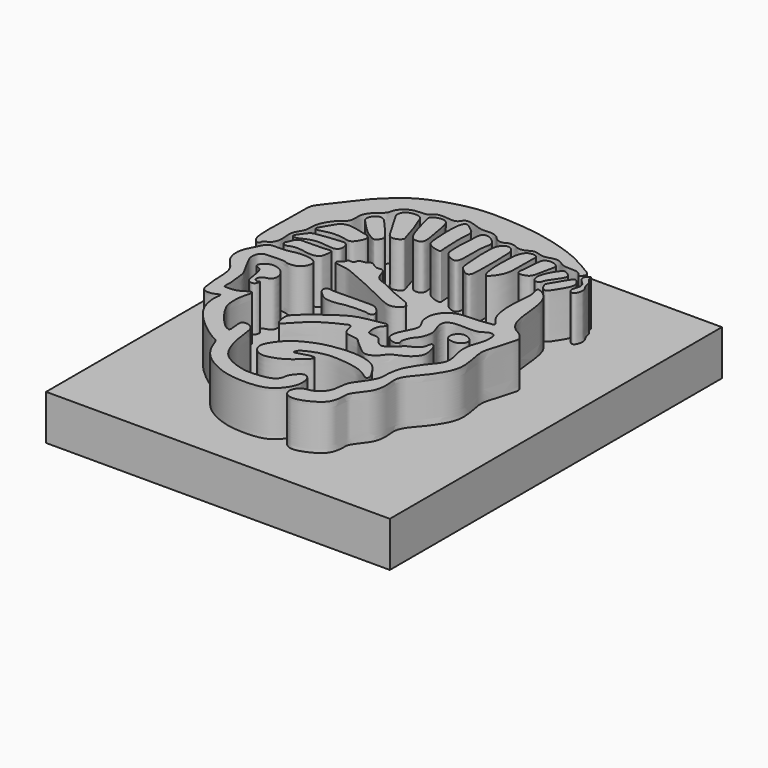
from build123d import *

# Parameters (mm, degrees)
F1_DEPTH = 25.4
F2_W     = 96.9264013693
F2_H     = 117.0432046056
F3_DEPTH = 12.7


with BuildPart() as f1:
    # F0 (on Top) → F1 (new body)
    with BuildSketch(Plane.XY):
        with BuildLine():
            add(Edge.make_bspline(
                [(-40.2134470642, -13.6436549947), (-40.5038319253, -13.0532989312), (-40.9712662134, -12.0357692788), (-40.3828119426, -9.0838404135), (-37.4700159523, -9.1659597907), (-33.6801272021, -8.8772320002), (-32.7655772786, -9.6282652278), (-29.8023894039, -9.4210274483), (-28.3806589854, -7.5498569946), (-28.0532124759, -5.5301169959), (-29.9501063345, -4.2010879959), (-33.9584884018, -4.060553572), (-36.4882191847, -4.9901386676), (-39.7344326102, -4.8370794081), (-41.852988261, -5.0813649106), (-43.0611123611, -7.9930232863), (-44.6638586961, -10.8148641524), (-44.6805787942, -13.9824924027), (-43.4351839453, -16.5508592113), (-41.4060540395, -18.327504016), (-40.4817112793, -20.4170340166), (-40.2150456125, -23.173487216), (-40.2371317705, -25.6148272624), (-39.7897618651, -28.8111673703), (-39.4242040094, -31.1359618698), (-36.7206525589, -31.2192672972), (-35.6066458214, -30.6210898454), (-34.4127301406, -30.0990799373), (-34.932395965, -32.2774129262), (-34.6889736884, -34.3855625988), (-33.9514081898, -37.3805205335), (-31.9389951827, -40.3046677573), (-29.0667186094, -43.1618199647), (-26.052819601, -45.5593423485), (-23.5900655555, -47.2267415521), (-21.6999075012, -47.8249153248), (-21.0648357224, -50.7700427907), (-18.8106721799, -54.2710823292), (-15.7050192032, -56.747814972), (-10.9850909536, -58.9656562044), (-5.5210704614, -59.6254274225), (0.0655429157, -59.2721168152), (3.1418643476, -57.3279514264), (5.3379892447, -54.0854350072), (5.6011670768, -51.5204836423), (5.2429584174, -49.3374778631), (3.4009534995, -48.166607769), (1.8703771285, -49.6207679802), (0.6615174644, -51.2282183426), (0.7409672686, -52.993382624), (-0.928557497, -54.7108114083), (-4.556009372, -55.1621405529), (-8.4581184608, -55.3892312796), (-13.3437110299, -53.5718738684), (-15.8033997352, -51.6433831739), (-17.4804730559, -48.8032608251), (-18.6647319579, -44.6349468246), (-19.0353626337, -40.8983524571), (-19.4757454842, -38.3228496413), (-21.5701928172, -37.2608658786), (-23.1594355454, -37.7347875195), (-22.9633855567, -39.5685823373), (-22.5875095291, -42.186811965), (-23.232268811, -42.0865318242), (-24.1233688412, -41.7328370024), (-25.2311286943, -40.8741082801), (-28.213025083, -37.5769037551), (-30.2068242336, -34.1381189549), (-30.7460865655, -32.4917857606), (-30.7936590907, -28.9726861151), (-30.1021813845, -26.3503756002), (-29.7493093459, -25.166157434), (-30.5926807443, -24.9813323567), (-31.6427370917, -25.773252658), (-33.4709586463, -26.8433998571), (-36.2557679667, -26.8237017314), (-36.7498527526, -26.6771194484), (-36.4617540337, -24.7653587113), (-37.0026261542, -21.1625112292), (-37.1052353815, -19.1935704677), (-38.8213673131, -16.3662075654), (-39.8354152195, -14.4121984746), (-40.2134470642, -13.6436549947)],
                knots=[0, 0, 0, 0, 0.0105854357, 0.0227038139, 0.0355615522, 0.0506964042, 0.0590934994, 0.0718715099, 0.08372586, 0.0940838712, 0.1051368075, 0.1206855449, 0.1338879249, 0.147872312, 0.1586917055, 0.1720366682, 0.1864080274, 0.2000583123, 0.2131788584, 0.2259198188, 0.2376677544, 0.2505637198, 0.2630490339, 0.2772986456, 0.2884688624, 0.3002440343, 0.3096215137, 0.3164567212, 0.3264983543, 0.3384916292, 0.3520782106, 0.3668620136, 0.3827581289, 0.3983550294, 0.4118200351, 0.4221569994, 0.4351815037, 0.4512043984, 0.4668630146, 0.4845956824, 0.503265583, 0.5216125929, 0.5364037424, 0.5516107261, 0.5641673247, 0.5755537169, 0.5858159785, 0.5965098416, 0.6076312106, 0.6176334598, 0.6290166971, 0.6438033901, 0.6596293721, 0.6773473823, 0.691109071, 0.7051053782, 0.7215553422, 0.7369683211, 0.7492434926, 0.7605774012, 0.769367475, 0.7798612926, 0.7919744263, 0.7966216104, 0.8041149769, 0.8133299168, 0.8300412854, 0.8457482662, 0.8560105345, 0.8706321915, 0.8839702758, 0.8916090014, 0.8975101119, 0.9062586889, 0.9181242245, 0.9309764693, 0.9355028424, 0.9456931412, 0.9609607679, 0.972097378, 0.9862195579, 1, 1, 1, 1], degree=3))
        make_face()
        with BuildLine():
            add(Edge.make_bspline(
                [(-36.9890481234, 1.9141569501), (-37.6086093115, 1.6183880837), (-38.5317237833, 1.0516364801), (-40.4055938126, 1.3458247704), (-38.8954202479, 3.4409428718), (-37.7142225728, 5.0654187852), (-36.2422882152, 5.4533680411), (-31.0847105816, 6.0055868791), (-29.4042524296, 6.2039104022), (-28.1776089982, 6.0259950489), (-27.4019390923, 3.5957598157), (-28.6162726688, 2.2319888659), (-30.9662986649, 2.5583398946), (-34.3116035087, 2.9699572864), (-36.2321994637, 2.2754647181), (-36.9890481234, 1.9141569501)],
                knots=[0, 0, 0, 0, 0.072612367, 0.129661764, 0.2048222141, 0.2807607212, 0.345890099, 0.4667093526, 0.5374814039, 0.5905759148, 0.6694874813, 0.7336228202, 0.8127819433, 0.9112975866, 1, 1, 1, 1], degree=3))
        make_face()
    extrude(amount=F1_DEPTH)



with BuildPart() as f1b:
    # F0 (on Top) → F1, piece 2 (new body)
    with BuildSketch(Plane.XY):
        with BuildLine():
            add(Edge.make_bspline(
                [(-35.3266075253, -16.0623975098), (-35.4972584298, -15.6958523644), (-35.9577022635, -15.0490288372), (-37.1653320579, -14.8763550547), (-37.4622378024, -13.8763719918), (-35.9694428669, -12.2011305597), (-33.6958844721, -12.0077739228), (-31.3642934169, -13.1003837915), (-29.9891050699, -15.3295362371), (-30.5140421494, -17.6267172637), (-32.215666586, -17.7794257093), (-33.1899626709, -18.4639808352), (-33.6363150575, -19.8373776846), (-32.2927485056, -20.601676247), (-31.836702742, -19.6812009092), (-31.7990430425, -21.0156581463), (-32.6426422962, -21.8861025724), (-34.3389047052, -21.358790101), (-34.6550812728, -19.4363616515), (-34.8919011587, -17.4700956508), (-35.1363620882, -16.471030219), (-35.3266075253, -16.0623975098)],
                knots=[0, 0, 0, 0, 0.0473231751, 0.0931074818, 0.1316273518, 0.193737266, 0.2588862114, 0.3280781791, 0.3976259368, 0.4589092763, 0.5125312499, 0.5600258653, 0.6082496238, 0.6549574763, 0.6858732626, 0.7261825163, 0.7726873443, 0.8248430499, 0.8843108095, 0.9472430682, 1, 1, 1, 1], degree=3))
        make_face()
    extrude(amount=F1_DEPTH)


with BuildPart() as f1c:
    # F0 (on Top) → F1, piece 3 (new body)
    with BuildSketch(Plane.XY):
        with BuildLine():
            add(Edge.make_bspline(
                [(-12.175809592, -13.3968461305), (-13.962078305, -13.4377839428), (-16.476435339, -13.5444627063), (-18.4696160942, -13.0990432929), (-18.9677203075, -14.6996565823), (-17.4880204322, -16.1364312172), (-15.7339827969, -17.7820473891), (-11.7939436123, -17.5276038721), (-10.3801314326, -16.9095088093), (-4.0682803098, -16.6837951327), (-3.6200768269, -17.3062140897), (-1.6812831301, -16.6008245729), (-4.2750977921, -13.3880830635), (-6.4565823701, -13.3288982131), (-10.1699988377, -13.3508768407), (-12.175809592, -13.3968461305)],
                knots=[0, 0, 0, 0, 0.1027704203, 0.1643350092, 0.2158170795, 0.2823859054, 0.3574579932, 0.4477449421, 0.5161774552, 0.6330677274, 0.6739522117, 0.7262824172, 0.8116726581, 0.8845985417, 1, 1, 1, 1], degree=3))
        make_face()
    extrude(amount=F1_DEPTH)


with BuildPart() as f1d:
    # F0 (on Top) → F1, piece 4 (new body)
    with BuildSketch(Plane.XY):
        with BuildLine():
            add(Edge.make_bspline(
                [(0, -40.7434217632), (0.2550089068, -40.8908280021), (0.0572282511, -41.8183311028), (-1.4831668381, -43.1030839423), (-4.0909554186, -45.4202079261), (-6.9829014151, -46.7046233332), (-10.7214378432, -47.5300746976), (-13.3893377622, -44.5219611327), (-12.1320019639, -41.3716536873), (-9.141106404, -37.6526166601), (-4.7511540043, -35.5585671529), (-2.2082004905, -34.6484818562), (1.6787778646, -33.9443538732), (5.7403798443, -33.6588574681), (9.9736766295, -34.376182303), (12.7629735747, -35.8806397687), (14.5269699842, -38.6402080561), (15.6656685159, -40.6177857059), (14.9915137008, -41.6993435417), (12.9071145673, -39.7743634452), (9.9757950754, -38.6694389514), (4.8867949575, -37.9685461739), (0.7319416308, -37.9294166922), (-4.0505929199, -39.7494504251), (-5.0513016798, -40.8892973736), (-5.2166015657, -41.8677113849), (-3.8359844809, -41.4940385204), (-0.5534711144, -40.4234913877), (0, -40.7434217632)],
                knots=[0, 0, 0, 0, 0.0206705355, 0.0529636374, 0.0950381864, 0.1358320371, 0.1781274716, 0.2185821362, 0.2576980575, 0.3072862008, 0.3564718581, 0.3936610023, 0.4377324292, 0.4839787069, 0.5302887211, 0.5698482529, 0.6109457689, 0.6439968083, 0.662486097, 0.6967267402, 0.7381146551, 0.7885277067, 0.8361118954, 0.8860866204, 0.9130842841, 0.9304810607, 0.9551366874, 1, 1, 1, 1], degree=3))
        make_face()
    extrude(amount=F1_DEPTH)


with BuildPart() as f1e:
    # F0 (on Top) → F1, piece 5 (new body)
    with BuildSketch(Plane.XY):
        with BuildLine():
            add(Edge.make_bspline(
                [(10.481367819, -52.9852025211), (10.1057038761, -53.2334762501), (9.3868343996, -53.6432463166), (7.105318589, -53.7802271793), (5.5379589581, -55.6953176891), (5.621418715, -57.9573159548), (8.2637918782, -59.4847403613), (12.6896903935, -57.7699512925), (15.4590722349, -55.8533247572), (16.4777159072, -53.6765375233), (16.7130225112, -51.1308906631), (16.5406671551, -49.7112398527), (18.7594635754, -46.8016379905), (20.3710932001, -44.6987023232), (20.9134433349, -41.0598633774), (20.2139722514, -37.9243135115), (21.5514648548, -35.1561540011), (23.9057813731, -32.6703413651), (26.6572085071, -28.8791360661), (28.44402102, -24.9429116068), (28.0853493643, -21.0336360459), (27.3534834554, -17.6007602298), (27.1204363152, -14.9322526668), (28.6143454232, -11.1154652758), (29.2701283527, -7.7451513556), (30.1299822693, -5.6994795216), (28.1143512178, -3.6252370906), (26.1813913382, -2.8537382587), (23.9501923858, -0.0029204504), (23.4225417353, 5.2670723981), (22.9004855358, 10.0125319135), (21.8018431376, 13.0906988334), (20.0139764252, 14.7493807415), (18.1497923111, 15.5030064107), (18.131500048, 14.6036296701), (18.8946148473, 12.7855586038), (18.4185250801, 8.8222478367), (18.1474952384, 4.1732985388), (18.8864235142, -0.597449726), (20.5373536115, -2.6725041874), (21.6372786424, -3.8990357185), (20.1399919421, -4.0960962659), (16.5068090043, -4.6685047846), (12.0351722124, -4.4786041784), (9.0928453674, -6.1028884328), (7.9090789163, -8.1059417154), (7.3845580799, -9.5557066185), (7.5479081613, -12.5333955357), (8.9953681272, -14.1892898252), (9.0575265732, -16.1339566967), (7.4373231239, -18.7826111354), (6.4010282834, -21.421636411), (6.8946371048, -23.3940237614), (9.2197972244, -24.553898415), (10.6122037289, -23.9028194683), (9.9925320776, -23.0348301568), (10.1959817003, -21.9536912939), (10.9405536832, -20.0013326602), (12.2295139, -18.9701448474), (13.5109525698, -15.3846240674), (11.9480867696, -12.6849278944), (11.6782242911, -9.9490466567), (13.761636726, -8.7576513151), (17.395892537, -8.9391852647), (21.0262448453, -8.9279169766), (22.3711096208, -7.3980710741), (24.3084708315, -7.5152866295), (24.6400235615, -8.8318310453), (24.5881651741, -11.6956432838), (23.387850378, -14.3066653641), (22.9215598182, -17.1770768728), (23.6104774504, -20.6494143714), (24.2780823643, -22.830559414), (23.8281191951, -25.2949179696), (21.4040741934, -27.7652442841), (19.4333085282, -30.9014604063), (17.8868065814, -33.7532891971), (17.5149679315, -37.3212683357), (17.64144859, -39.8365725522), (15.0943359094, -43.416200313), (13.189371433, -45.9974479426), (13.2036608443, -49.3463892426), (12.1708587579, -51.7738008355), (10.9501389787, -52.6753948697), (10.481367819, -52.9852025211)],
                knots=[0, 0, 0, 0, 0.0083827011, 0.0193218471, 0.0305936986, 0.0409768384, 0.0528329038, 0.0689015669, 0.0825925137, 0.0939689897, 0.1056335827, 0.1144435458, 0.1282679574, 0.1407584262, 0.1547334716, 0.1680222102, 0.1805985307, 0.1944544627, 0.2106734319, 0.2260838738, 0.2407486113, 0.2546422286, 0.2667296087, 0.2817888379, 0.2958082047, 0.3062368459, 0.3180285776, 0.3288796174, 0.3424622186, 0.3597520556, 0.3762702317, 0.3894814131, 0.4013294934, 0.4106653838, 0.4159670691, 0.4262117298, 0.4410660624, 0.4575884512, 0.4738300757, 0.486133142, 0.4940032114, 0.5012347596, 0.5158522949, 0.5318851351, 0.5452093438, 0.5562003475, 0.5654915708, 0.5780602435, 0.588939414, 0.5987631866, 0.6119479309, 0.6244733398, 0.6345291421, 0.6461212625, 0.653896109, 0.6604373475, 0.6682403283, 0.6787810166, 0.6884906317, 0.7023451351, 0.7155850518, 0.7270883763, 0.7375437069, 0.7520224707, 0.7660452794, 0.7762899371, 0.7855430438, 0.7934785232, 0.8060212899, 0.8187541103, 0.8314573892, 0.8454324314, 0.8566790031, 0.8679508565, 0.8817615911, 0.8962077018, 0.9097167081, 0.9235790615, 0.9353603428, 0.9506875999, 0.9641610261, 0.9775228146, 0.9895396708, 1, 1, 1, 1], degree=3))
        make_face()
    extrude(amount=F1_DEPTH)


with BuildPart() as f1f:
    # F0 (on Top) → F1, piece 6 (new body)
    with BuildSketch(Plane.XY):
        with BuildLine():
            add(Edge.make_bspline(
                [(17.4907818437, -15.4700446874), (17.1151979262, -15.1544877651), (16.7158787145, -13.9380716767), (17.5094432987, -12.3221218095), (19.0726581308, -11.5663291244), (21.1671954012, -12.2918146022), (22.3917264893, -14.2009770312), (20.2838849914, -16.0491594903), (18.8723018315, -15.8604322291), (17.8433708452, -15.766281813), (17.4907818437, -15.4700446874)],
                knots=[0, 0, 0, 0, 0.1198463059, 0.2434983858, 0.3630205508, 0.5010414267, 0.6294366117, 0.7731817435, 0.8874912173, 1, 1, 1, 1], degree=3))
        make_face()
    extrude(amount=F1_DEPTH)


with BuildPart() as f1g:
    # F0 (on Top) → F1, piece 7 (new body)
    with BuildSketch(Plane.XY):
        with BuildLine():
            add(Edge.make_bspline(
                [(13.2950088009, -23.61478284), (13.8348931255, -23.3719104476), (15.125243671, -22.8351532415), (16.0326731284, -21.2276110646), (16.0416305597, -19.65010325), (17.2120550863, -19.6877070955), (18.2160433992, -22.7492744313), (18.2563774038, -25.3331510511), (15.9850869785, -27.5837265934), (13.7395188615, -28.5317025479), (11.7239932549, -29.3735631459), (10.6986449854, -31.4171037153), (7.8082291311, -33.1191705401), (5.3238765118, -31.1331587477), (2.9044288788, -29.0002456724), (1.786599307, -27.6694713139), (-1.4178519176, -27.8441265379), (-2.5642456075, -26.3711474512), (-2.8259560494, -23.5115455616), (-4.5760845795, -24.296530775), (-7.3188478304, -25.527596382), (-11.948728853, -28.3970124143), (-15.0116932785, -32.24535168), (-16.307971164, -33.189493036), (-16.9713594686, -31.6407063527), (-17.1819559941, -29.9154185107), (-16.9400214355, -28.4563498107), (-13.8527577015, -25.7304982924), (-9.6648673277, -22.5663788095), (-5.1834985564, -19.5799945508), (0.3983263813, -18.8666301065), (2.8805340601, -18.244482919), (3.1467245055, -19.0755055974), (2.5225906957, -19.9690656397), (1.8622895301, -20.6486046658), (1.5592825514, -22.6572749998), (2.0098491605, -24.4534072576), (3.7626807349, -24.3560217497), (5.4176067955, -24.5638185498), (6.4976419148, -26.4557408647), (8.0617079498, -27.5626666188), (9.6414305671, -26.5253748059), (11.1979381079, -25.3126103162), (12.1010874827, -24.1823941472), (12.8503587562, -23.814813134), (13.2950088009, -23.61478284)],
                knots=[0, 0, 0, 0, 0.0218070593, 0.0431234208, 0.061254979, 0.0738721666, 0.1010596607, 0.1265183506, 0.1534633819, 0.1783036334, 0.2007273221, 0.2242850447, 0.2508267707, 0.277679895, 0.3060360971, 0.3262907215, 0.3528344392, 0.3738360917, 0.3976600759, 0.4152419551, 0.4427929972, 0.4802820701, 0.515422649, 0.5316137453, 0.54957411, 0.5706398277, 0.5887713891, 0.6197287143, 0.6564767345, 0.6931486701, 0.7308974522, 0.7538600161, 0.7653274163, 0.7811833671, 0.796580367, 0.8188030539, 0.8385548701, 0.857825069, 0.8775962114, 0.9003812732, 0.920640384, 0.9410194366, 0.9634563401, 0.9820396528, 1, 1, 1, 1], degree=3))
        make_face()
    extrude(amount=F1_DEPTH)


with BuildPart() as f1h:
    # F0 (on Top) → F1, piece 8 (new body)
    with BuildSketch(Plane.XY):
        with BuildLine():
            add(Edge.make_bspline(
                [(-6.005553063, -5.5482722819), (-4.2626675229, -6.3525546424), (-0.6960493656, -7.5363531897), (-0.0735943929, -8.2951825559), (0.9376558196, -9.3703830611), (-0.7556190983, -10.8294300332), (-2.815800733, -11.4188731389), (-5.9541970542, -9.9006417242), (-12.0277826397, -6.9213939985), (-17.7209732591, -4.4389249739), (-21.3001847011, -2.9222257695), (-24.8504041533, -3.0054633078), (-24.5478163437, -1.5600209245), (-23.0949665475, -0.9596880534), (-23.0749253321, 0.3449919826), (-21.3198555493, -0.4619385045), (-21.3809135653, 1.6082161882), (-19.3424176116, 1.314974933), (-18.4204110876, 2.6812743144), (-16.8433754716, 1.5036862348), (-15.8366504443, 0.9508758634), (-14.5310556941, 1.4151149864), (-13.4558582135, 0.5293829858), (-12.9386926309, -2.8478756676), (-9.2209924876, -3.6319082935), (-7.4570856434, -4.8784393966), (-6.005553063, -5.5482722819)],
                knots=[0, 0, 0, 0, 0.0667185024, 0.0948163333, 0.123780369, 0.1615582908, 0.2015477576, 0.2521917791, 0.3261137412, 0.3965827167, 0.4533780597, 0.5008285532, 0.5265947447, 0.5609772307, 0.5872793164, 0.6177890861, 0.6498340525, 0.6857406118, 0.7177514598, 0.7535847027, 0.783947757, 0.8145103578, 0.8446561246, 0.8934268482, 0.94443463, 1, 1, 1, 1], degree=3))
        make_face()
    extrude(amount=F1_DEPTH)


with BuildPart() as f1i:
    # F0 (on Top) → F1, piece 9 (new body)
    with BuildSketch(Plane.XY):
        with BuildLine():
            add(Edge.make_bspline(
                [(-40.9538783133, 0.7207064773), (-40.8926457501, -0.1425373131), (-40.6044174786, -1.9953952776), (-41.8152417336, -4.2210841827), (-43.7057223087, -4.5771993127), (-43.3172967931, -6.0679911849), (-45.7660667091, -5.2647503656), (-46.0519791054, 0.4491609292), (-45.7213378873, 6.5723176219), (-45.7869960383, 13.7474246169), (-45.4454218071, 15.8377628901), (-41.4351894324, 20.5046647967), (-37.558420593, 26.0633493644), (-33.6966086012, 29.4755162368), (-30.0794225513, 32.5134000531), (-22.9336113137, 35.4833019443), (-15.4008533066, 37.1053297264), (-8.6599092462, 37.0876502228), (1.8589268769, 36.3718796817), (12.0104013583, 33.4624153703), (17.0363686159, 31.0738862185), (20.6791774698, 28.7996943774), (22.8037855099, 27.6442850863), (21.2463162651, 25.4524071909), (20.438247231, 26.9734651559), (19.2169203835, 27.4469555413), (16.9327100454, 27.3567743987), (15.0539782676, 27.643895653), (13.7496087082, 28.943796319), (11.5564719547, 28.9411759616), (10.0962748471, 28.2196116149), (8.2313558821, 28.3554561494), (6.8743124711, 29.0350237755), (5.4279824976, 28.616999582), (4.3996061322, 27.8497454849), (2.4384634582, 27.6351464056), (1.4950822459, 28.4485393338), (-0.5908711322, 28.6450106123), (-1.6483997631, 27.5726713152), (-3.6630245324, 27.9407635636), (-4.5037535998, 29.2833323734), (-6.3047594809, 30.0206885245), (-8.1845335047, 29.7327080381), (-9.978958417, 29.831445458), (-12.1422304034, 30.8169826757), (-15.0459435858, 31.327053125), (-15.5926876562, 29.2838587013), (-17.6690150311, 29.1708395097), (-19.3271561603, 29.5730491774), (-22.1066827156, 29.2905542773), (-22.6436270006, 27.8168220266), (-25.328058942, 27.7400563044), (-27.502894336, 27.5463790179), (-29.7716420166, 25.6901316021), (-30.2452005374, 24.1022969814), (-30.5476857531, 22.8557552484), (-32.1715798462, 21.8432752016), (-33.6147585456, 20.2255978792), (-34.556255383, 18.4344065338), (-34.2274091625, 16.2412271787), (-34.822226235, 14.3691602395), (-36.4610865416, 13.5749807342), (-38.2578538125, 11.1422562052), (-39.3132687146, 8.786990468), (-39.2156490247, 6.1330014548), (-39.6797820972, 4.7029208663), (-40.9782596996, 2.8608620157), (-41.0081326566, 1.4855727923), (-40.9538783133, 0.7207064773)],
                knots=[0, 0, 0, 0, 0.0154472407, 0.02980268, 0.0415671016, 0.0502708959, 0.0615166443, 0.0829898223, 0.1076886549, 0.1321565176, 0.1455300408, 0.1681351996, 0.1931823625, 0.2141279271, 0.2342777856, 0.2602466454, 0.2862216805, 0.3104238427, 0.3410352879, 0.371603016, 0.3937639847, 0.4131852959, 0.4260551316, 0.4380222693, 0.4481037983, 0.4588052309, 0.4729376868, 0.4857519986, 0.4980711047, 0.5114150297, 0.5234231283, 0.5359291591, 0.5473525715, 0.558305972, 0.5690946174, 0.5816126559, 0.5920429479, 0.6048906606, 0.6160358439, 0.628447007, 0.6400702321, 0.652699489, 0.6655405409, 0.6778847269, 0.692699457, 0.707578865, 0.719479568, 0.7319225986, 0.7447968492, 0.7596418641, 0.7702969364, 0.784825714, 0.7990847842, 0.8145929204, 0.8265019966, 0.8366562049, 0.8493041079, 0.8632129919, 0.8762854303, 0.8901025045, 0.9026085423, 0.9148998715, 0.9310079486, 0.9462918168, 0.9611883294, 0.9726650141, 0.9863131665, 1, 1, 1, 1], degree=3))
        make_face()
    extrude(amount=F1_DEPTH)


with BuildPart() as f1j:
    # F0 (on Top) → F1, piece 10 (new body)
    with BuildSketch(Plane.XY):
        with BuildLine():
            add(Edge.make_bspline(
                [(-38.979396224, -1.3525033137), (-38.6977461323, -0.7837733775), (-38.2661277475, 0.9654593973), (-35.7444748266, 1.0636889939), (-30.4951994353, 0.8874526095), (-28.3825360852, 1.5771914364), (-28.5861066144, -0.8127057471), (-28.9758882763, -2.7511398238), (-31.6131253169, -3.0567106399), (-33.4198420175, -2.5971408515), (-36.6481096787, -2.1953047559), (-38.2209429355, -3.417474635), (-39.6550072998, -2.2842098949), (-39.1738366988, -1.7451327572), (-38.979396224, -1.3525033137)],
                knots=[0, 0, 0, 0, 0.0831365492, 0.1697354908, 0.304730039, 0.3768819454, 0.454522798, 0.5328335274, 0.6185110589, 0.7006152792, 0.8018786407, 0.8788318086, 0.9426056992, 1, 1, 1, 1], degree=3))
        make_face()
    extrude(amount=F1_DEPTH)


with BuildPart() as f1k:
    # F0 (on Top) → F1, piece 11 (new body)
    with BuildSketch(Plane.XY):
        with BuildLine():
            add(Edge.make_bspline(
                [(-34.2461764812, 7.7818217687), (-35.2521283016, 7.6376750731), (-36.6063377913, 7.0996382436), (-38.9711294628, 6.9521737104), (-36.3753668963, 10.5317691924), (-35.6610281586, 12.335328408), (-33.2652369867, 13.5478196735), (-29.2379108841, 12.221876975), (-27.1766482556, 12.0327867228), (-26.0951526332, 10.8742979235), (-26.8648895195, 9.0694492728), (-28.2246555576, 6.946427194), (-30.4811050493, 7.8198321053), (-33.0519555323, 7.9529462701), (-34.2461764812, 7.7818217687)],
                knots=[0, 0, 0, 0, 0.0892904545, 0.1502018209, 0.2504188524, 0.3305928242, 0.4126270262, 0.5237733144, 0.6019749636, 0.6616012768, 0.7352670352, 0.8155419176, 0.8939983713, 1, 1, 1, 1], degree=3))
        make_face()
    extrude(amount=F1_DEPTH)


with BuildPart() as f1l:
    # F0 (on Top) → F1, piece 12 (new body)
    with BuildSketch(Plane.XY):
        with BuildLine():
            add(Edge.make_bspline(
                [(-31.3991419971, 16.4965186268), (-31.9220040857, 17.0321993888), (-32.7002296255, 17.7318076783), (-32.118324141, 19.7125770612), (-30.7228288945, 20.7306455349), (-29.1846516378, 20.3619037336), (-27.5780127179, 18.3949700923), (-23.3077945285, 13.6816504051), (-23.6115074982, 12.6331260394), (-24.5848178332, 10.9612410657), (-26.2083547859, 11.8908503981), (-28.4456439929, 13.2490905424), (-30.5669417119, 15.6439158228), (-31.3991419971, 16.4965186268)],
                knots=[0, 0, 0, 0, 0.0801429549, 0.1613243604, 0.2384901887, 0.3075386577, 0.4090056846, 0.5604723417, 0.6208242261, 0.69649426, 0.7701760641, 0.8724424828, 1, 1, 1, 1], degree=3))
        make_face()
    extrude(amount=F1_DEPTH)


with BuildPart() as f1m:
    # F0 (on Top) → F1, piece 13 (new body)
    with BuildSketch(Plane.XY):
        with BuildLine():
            add(Edge.make_bspline(
                [(-23.899640888, 15.871560201), (-24.9048990037, 17.5463241369), (-27.7270911465, 22.4348267628), (-28.5096531635, 23.8275654632), (-27.827650676, 25.8382154972), (-25.3146448299, 26.5509448422), (-23.3384326227, 26.0992260916), (-22.6027223491, 24.1732256501), (-21.03097312, 20.1851926664), (-20.0699970379, 16.4473972374), (-19.6352714528, 15.5717887119), (-20.7975401342, 14.4593126813), (-22.8594644257, 14.2018724225), (-23.3944588903, 15.0299250254), (-23.899640888, 15.871560201)],
                knots=[0, 0, 0, 0, 0.1491400667, 0.2184064027, 0.2891794002, 0.3742607922, 0.446750554, 0.5200614487, 0.6354814225, 0.7416051018, 0.7892956437, 0.8527797129, 0.9250512126, 1, 1, 1, 1], degree=3))
        make_face()
    extrude(amount=F1_DEPTH)


with BuildPart() as f1n:
    # F0 (on Top) → F1, piece 14 (new body)
    with BuildSketch(Plane.XY):
        with BuildLine():
            add(Edge.make_bspline(
                [(-19.3860530853, 18.4061154723), (-20.2913210482, 20.2896279669), (-21.5831905651, 25.7591270904), (-22.0610494114, 27.2998841687), (-19.931417181, 28.4108956268), (-17.432282711, 28.1352796155), (-16.6887170325, 25.3001408381), (-16.2678406753, 21.9940020159), (-15.4928635917, 18.7978044592), (-15.7439452779, 16.7921848663), (-17.9728814853, 16.5525956936), (-18.8899116631, 17.3738370684), (-19.3860530853, 18.4061154723)],
                knots=[0, 0, 0, 0, 0.1711752709, 0.2436111829, 0.330560066, 0.4213868249, 0.5197993603, 0.6350773131, 0.7474217894, 0.8263405213, 0.9061856314, 1, 1, 1, 1], degree=3))
        make_face()
    extrude(amount=F1_DEPTH)


with BuildPart() as f1o:
    # F0 (on Top) → F1, piece 15 (new body)
    with BuildSketch(Plane.XY):
        with BuildLine():
            add(Edge.make_bspline(
                [(-14.629425481, 23.6488226801), (-14.6810786676, 25.4970820354), (-14.6106826109, 28.6127633025), (-13.4112223622, 30.1976370094), (-11.5529974208, 28.5501786619), (-9.7999737346, 27.2598782017), (-10.41660567, 25.0155358117), (-10.0846518681, 17.2047663563), (-9.7563279336, 15.653361392), (-14.0203468268, 16.8524843316), (-14.3517806187, 19.3009400985), (-14.5812337388, 21.9244210695), (-14.629425481, 23.6488226801)],
                knots=[0, 0, 0, 0, 0.1329434766, 0.200029151, 0.2855891952, 0.3679441453, 0.4562234214, 0.6223120418, 0.6786539711, 0.7874209847, 0.8759654891, 1, 1, 1, 1], degree=3))
        make_face()
    extrude(amount=F1_DEPTH)


with BuildPart() as f1p:
    # F0 (on Top) → F1, piece 16 (new body)
    with BuildSketch(Plane.XY):
        with BuildLine():
            add(Edge.make_bspline(
                [(-8.3104008809, 21.3920287788), (-8.3530003435, 20.3669449132), (-8.2300376136, 18.2943591472), (-8.1604608184, 16.0725598954), (-5.7928418526, 14.5650994333), (-3.7281206885, 14.4769126808), (-3.9021051767, 19.0109140137), (-3.7124130661, 23.9344508913), (-3.0007443839, 25.6516885657), (-4.3810790993, 27.4502771729), (-6.1938646967, 28.3569235255), (-8.1156824702, 28.1275778691), (-7.9582563131, 24.265852467), (-8.2679786156, 22.4128486901), (-8.3104008809, 21.3920287788)],
                knots=[0, 0, 0, 0, 0.092173982, 0.1676843534, 0.2516105047, 0.313205266, 0.417266433, 0.536354792, 0.6032257467, 0.6768457976, 0.7514879532, 0.8125908876, 0.9082094263, 1, 1, 1, 1], degree=3))
        make_face()
    extrude(amount=F1_DEPTH)


with BuildPart() as f1q:
    # F0 (on Top) → F1, piece 17 (new body)
    with BuildSketch(Plane.XY):
        with BuildLine():
            add(Edge.make_bspline(
                [(-1.9219375681, 20.3504301608), (-1.9660284411, 21.3968267645), (-1.9219371188, 23.990642567), (-1.5722914648, 26.0777684582), (0.5204931515, 27.6716555328), (2.350301632, 25.9753291254), (2.4183922397, 24.0919982711), (2.6392033644, 19.1936024303), (2.4352263698, 13.8757761649), (2.437115288, 11.980479015), (1.4892719567, 10.784781524), (-0.3959828968, 12.2892623551), (-1.6382839424, 13.1945339235), (-1.6901187423, 18.1215341649), (-1.8857221701, 19.4909400454), (-1.9219375681, 20.3504301608)],
                knots=[0, 0, 0, 0, 0.0911123569, 0.1616595862, 0.2306746411, 0.2974090923, 0.3618113981, 0.4690337689, 0.5813359242, 0.6459694723, 0.6946811962, 0.7628224433, 0.8230510771, 0.9251620563, 1, 1, 1, 1], degree=3))
        make_face()
    extrude(amount=F1_DEPTH)


with BuildPart() as f1r:
    # F0 (on Top) → F1, piece 18 (new body)
    with BuildSketch(Plane.XY):
        with BuildLine():
            add(Edge.make_bspline(
                [(4.1193277575, 22.6072259247), (4.1783596805, 23.8320443529), (4.3051791852, 25.4615471598), (5.4265366746, 27.69677715), (8.1568344361, 27.7682180772), (8.475063767, 26.0577810385), (8.1142694819, 21.4306402248), (8.4936585995, 16.9218601105), (6.0356195484, 13.5829723411), (4.8881736145, 12.9903916102), (3.9200740793, 16.5164843058), (4.0325939322, 20.8076371226), (4.1193277575, 22.6072259247)],
                knots=[0, 0, 0, 0, 0.100068586, 0.186029265, 0.2705011368, 0.3376791587, 0.4623503256, 0.5895283683, 0.7029641763, 0.7527202813, 0.8529722425, 1, 1, 1, 1], degree=3))
        make_face()
    extrude(amount=F1_DEPTH)


with BuildPart() as f1s:
    # F0 (on Top) → F1, piece 19 (new body)
    with BuildSketch(Plane.XY):
        with BuildLine():
            add(Edge.make_bspline(
                [(9.743954055, 20.0726725161), (9.8610236187, 21.2499571915), (10.1114314186, 25.1730387885), (10.3845451271, 26.7770162905), (12.0703181741, 27.674811888), (14.8421295889, 26.7244769697), (14.1395391538, 24.2756705756), (13.4141581671, 19.4374271945), (12.153519985, 18.7731377139), (10.5468952106, 18.2867868944), (9.6051218859, 19.0336197564), (9.6909611586, 19.5397609473), (9.743954055, 20.0726725161)],
                knots=[0, 0, 0, 0, 0.1567200212, 0.245338896, 0.3341189013, 0.4396967184, 0.5440964555, 0.6962080511, 0.7756517884, 0.8622431316, 0.9290588639, 1, 1, 1, 1], degree=3))
        make_face()
    extrude(amount=F1_DEPTH)


with BuildPart() as f1t:
    # F0 (on Top) → F1, piece 20 (new body)
    with BuildSketch(Plane.XY):
        with BuildLine():
            add(Edge.make_bspline(
                [(14.3964225426, 20.524032414), (14.6430042521, 22.2170132414), (16.5450738758, 25.3125992074), (17.605323936, 25.8778158833), (19.7226826247, 24.5414361157), (19.2435743492, 22.671566189), (16.4448784381, 19.3041063308), (16.6424922045, 18.0350422189), (14.8216912729, 17.7113387783), (14.2229018533, 19.3326739758), (14.3964225426, 20.524032414)],
                knots=[0, 0, 0, 0, 0.1935736076, 0.2792825713, 0.398773628, 0.5097074974, 0.6856835969, 0.7716612819, 0.8637813571, 1, 1, 1, 1], degree=3))
        make_face()
    extrude(amount=F1_DEPTH)


with BuildPart() as f1u:
    # F0 (on Top) → F1, piece 21 (new body)
    with BuildSketch(Plane.XY):
        with BuildLine():
            add(Edge.make_bspline(
                [(18.1461740285, 18.6838768423), (18.6197505047, 19.608588064), (20.8384748158, 23.3693868615), (21.8602145922, 24.3900829753), (23.6064575312, 22.4733821126), (22.9894050515, 20.2179043674), (21.519917955, 17.9863291967), (19.9343431303, 15.2920469815), (18.3738282969, 16.7442796337), (17.8913773479, 18.0687959353), (17.9784210747, 18.3563203721), (18.1461740285, 18.6838768423)],
                knots=[0, 0, 0, 0, 0.1822476464, 0.2659334823, 0.3756297074, 0.4907849767, 0.6244453448, 0.7482430924, 0.8455685491, 0.9354432018, 1, 1, 1, 1], degree=3))
        make_face()
    extrude(amount=F1_DEPTH)


with BuildPart() as f1v:
    # F0 (on Top) → F1, piece 22 (new body)
    with BuildSketch(Plane.XY):
        with BuildLine():
            add(Edge.make_bspline(
                [(24.3610367179, 23.2321843505), (24.0399114898, 23.7583549933), (22.8060101121, 24.4860097684), (22.2421417785, 26.2030456838), (24.0401764333, 27.6439258789), (23.810114085, 25.719773764), (25.1961618788, 25.14478277), (25.291960512, 23.0119833089), (26.2397936695, 21.9071776305), (26.4598563789, 20.6745343616), (25.6452980772, 18.0384037215), (23.5765402192, 19.5563114761), (24.6853928284, 21.4648627705), (24.6615410827, 22.7398014388), (24.3610367179, 23.2321843505)],
                knots=[0, 0, 0, 0, 0.0928438803, 0.1759468343, 0.2533622776, 0.3240904749, 0.3999980914, 0.4920611029, 0.5694765593, 0.6444344756, 0.7397527679, 0.8204443778, 0.9131180336, 1, 1, 1, 1], degree=3))
        make_face()
    extrude(amount=F1_DEPTH)


with BuildPart() as f1_1:
    add(f1.part)

    add(f1b.part)  # F3 merges F1b

    add(f1c.part)  # F3 merges F1c

    add(f1d.part)  # F3 merges F1d

    add(f1e.part)  # F3 merges F1e

    add(f1f.part)  # F3 merges F1f

    add(f1g.part)  # F3 merges F1g

    add(f1h.part)  # F3 merges F1h

    add(f1i.part)  # F3 merges F1i

    add(f1j.part)  # F3 merges F1j

    add(f1k.part)  # F3 merges F1k

    add(f1l.part)  # F3 merges F1l

    add(f1m.part)  # F3 merges F1m

    add(f1n.part)  # F3 merges F1n

    add(f1o.part)  # F3 merges F1o

    add(f1p.part)  # F3 merges F1p

    add(f1q.part)  # F3 merges F1q

    add(f1r.part)  # F3 merges F1r

    add(f1s.part)  # F3 merges F1s

    add(f1t.part)  # F3 merges F1t

    add(f1u.part)  # F3 merges F1u

    add(f1v.part)  # F3 merges F1v
    # F2 (on Top) → F3 (join)
    with BuildSketch(Plane.XY):
        with Locations((-2.5908029638, -12.9540003836)):
            Rectangle(F2_W, F2_H)
    extrude(amount=F3_DEPTH)


solid = f1_1.part
